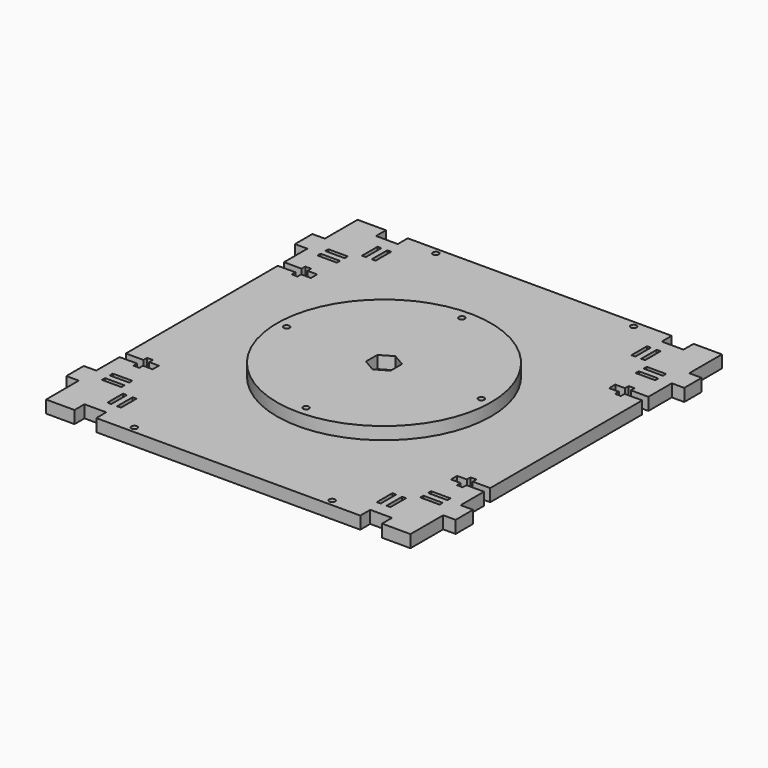
from build123d import *

# Parameters (mm, degrees)
F0_R     = 55
F0_R_2   = 1.5
F0_R_3   = 45
F1_DEPTH = 6.4
F2_DEPTH = 6
F0_R_4   = 85
F3_DEPTH = 6
F0_W     = 2
F0_H     = 10
F0_W_2   = 10
F0_H_2   = 2
F4_DEPTH = 6.4


with BuildPart() as f1:
    # F0 (on Top) → F1 (new body)
    with BuildSketch(Plane.XY):
        Circle(F0_R)
        with Locations((0, -50)):
            Circle(F0_R_2, mode=Mode.SUBTRACT)
        with Locations((-50, 0)):
            Circle(F0_R_2, mode=Mode.SUBTRACT)
        Circle(F0_R_3, mode=Mode.SUBTRACT)
        with Locations((50, 0)):
            Circle(F0_R_2, mode=Mode.SUBTRACT)
        with Locations((0, 50)):
            Circle(F0_R_2, mode=Mode.SUBTRACT)
        Circle(F0_R_3)
        Polygon((-6.35, 3.6661742094), (0, 7.3323484187), (6.35, 3.6661742094), (6.35, -3.6661742094), (0, -7.3323484187), (-6.35, -3.6661742094), align=None, mode=Mode.SUBTRACT)
    extrude(amount=F1_DEPTH)


with BuildPart() as f2:
    # F0 (on Top) → F2 (new body)
    with BuildSketch(Plane.XY):
        Circle(F0_R)
        with Locations((0, -50)):
            Circle(F0_R_2, mode=Mode.SUBTRACT)
        with Locations((-50, 0)):
            Circle(F0_R_2, mode=Mode.SUBTRACT)
        Circle(F0_R_3, mode=Mode.SUBTRACT)
        with Locations((50, 0)):
            Circle(F0_R_2, mode=Mode.SUBTRACT)
        with Locations((0, 50)):
            Circle(F0_R_2, mode=Mode.SUBTRACT)
    extrude(amount=F2_DEPTH)


with BuildPart() as f3:
    # F0 (on Top) → F3 (new body)
    with BuildSketch(Plane.XY):
        Circle(F0_R_4)
        Circle(F0_R, mode=Mode.SUBTRACT)
        Circle(F0_R)
        with Locations((0, -50)):
            Circle(F0_R_2, mode=Mode.SUBTRACT)
        with Locations((-50, 0)):
            Circle(F0_R_2, mode=Mode.SUBTRACT)
        Circle(F0_R_3, mode=Mode.SUBTRACT)
        with Locations((50, 0)):
            Circle(F0_R_2, mode=Mode.SUBTRACT)
        with Locations((0, 50)):
            Circle(F0_R_2, mode=Mode.SUBTRACT)
    extrude(amount=F3_DEPTH)


with BuildPart() as f4:
    # F0 (on Top) → F4 (new body)
    with BuildSketch(Plane.XY):
        Polygon((93.6, 78.994885087), (93.6, 100), (78.994885087, 100), (78.994885087, 93.6), (67.8103417158, 93.6), (67.8103417158, 100), (-67.8103417158, 100), (-67.8103417158, 93.6), (-78.994885087, 93.6), (-78.994885087, 100), (-93.6, 100), (-93.6, 78.994885087), (-100, 78.994885087), (-100, 67.8103417158), (-93.6, 67.8103417158), (-93.6, 52.7854223251), (-84.5765625, 52.7854223251), (-84.5765625, 55.1510473251), (-81.6, 55.1510473251), (-81.6, 52.7854223251), (-76.6, 52.7854223251), (-76.6, 48.7854223251), (-81.6, 48.7854223251), (-81.6, 46.4197973251), (-84.5765625, 46.4197973251), (-84.5765625, 48.7854223251), (-93.6, 48.7854223251), (-93.6, -48.7854223251), (-84.5765625, -48.7854223251), (-84.5765625, -46.4197973251), (-81.6, -46.4197973251), (-81.6, -48.7854223251), (-76.6, -48.7854223251), (-76.6, -52.7854223251), (-81.6, -52.7854223251), (-81.6, -55.1510473251), (-84.5765625, -55.1510473251), (-84.5765625, -52.7854223251), (-93.6, -52.7854223251), (-93.6, -67.8103417158), (-100, -67.8103417158), (-100, -78.994885087), (-93.6, -78.994885087), (-93.6, -100), (-78.994885087, -100), (-78.994885087, -93.6), (-67.8103417158, -93.6), (-67.8103417158, -100), (67.8103417158, -100), (67.8103417158, -93.6), (78.994885087, -93.6), (78.994885087, -100), (93.6, -100), (93.6, -78.994885087), (100, -78.994885087), (100, -67.8103417158), (93.6, -67.8103417158), (93.6, -52.7854223251), (84.5765625, -52.7854223251), (84.5765625, -55.1510473251), (81.6, -55.1510473251), (81.6, -52.7854223251), (76.6, -52.7854223251), (76.6, -48.7854223251), (81.6, -48.7854223251), (81.6, -46.4197973251), (84.5765625, -46.4197973251), (84.5765625, -48.7854223251), (93.6, -48.7854223251), (93.6, 48.7854223251), (84.5765625, 48.7854223251), (84.5765625, 46.4197973251), (81.6, 46.4197973251), (81.6, 48.7854223251), (76.6, 48.7854223251), (76.6, 52.7854223251), (81.6, 52.7854223251), (81.6, 55.1510473251), (84.5765625, 55.1510473251), (84.5765625, 52.7854223251), (93.6, 52.7854223251), (93.6, 67.8103417158), (100, 67.8103417158), (100, 78.994885087), align=None)
        with Locations((-50.7854223251, -96.8)):
            Circle(F0_R_2, mode=Mode.SUBTRACT)
        with Locations((-71.6977112889, -81.7467170954)):
            Rectangle(F0_W, F0_H, mode=Mode.SUBTRACT)
        with Locations((-66.6977112889, -81.7467170954)):
            Rectangle(F0_W, F0_H, mode=Mode.SUBTRACT)
        with Locations((-81.7467170954, -71.6977112889)):
            Rectangle(F0_W_2, F0_H_2, mode=Mode.SUBTRACT)
        with Locations((-81.7467170954, -66.6977112889)):
            Rectangle(F0_W_2, F0_H_2, mode=Mode.SUBTRACT)
        with Locations((50.7854223251, -96.8)):
            Circle(F0_R_2, mode=Mode.SUBTRACT)
        with Locations((66.6977112889, -81.7467170954)):
            Rectangle(F0_W, F0_H, mode=Mode.SUBTRACT)
        with Locations((71.6977112889, -81.7467170954)):
            Rectangle(F0_W, F0_H, mode=Mode.SUBTRACT)
        with Locations((81.7467170954, -71.6977112889)):
            Rectangle(F0_W_2, F0_H_2, mode=Mode.SUBTRACT)
        with Locations((81.7467170954, -66.6977112889)):
            Rectangle(F0_W_2, F0_H_2, mode=Mode.SUBTRACT)
        with Locations((-81.7467170954, 66.6977112889)):
            Rectangle(F0_W_2, F0_H_2, mode=Mode.SUBTRACT)
        with Locations((-81.7467170954, 71.6977112889)):
            Rectangle(F0_W_2, F0_H_2, mode=Mode.SUBTRACT)
        with Locations((-71.6977112889, 81.7467170954)):
            Rectangle(F0_W, F0_H, mode=Mode.SUBTRACT)
        with Locations((-66.6977112889, 81.7467170954)):
            Rectangle(F0_W, F0_H, mode=Mode.SUBTRACT)
        with Locations((-50.7854223251, 96.8)):
            Circle(F0_R_2, mode=Mode.SUBTRACT)
        Circle(F0_R_4, mode=Mode.SUBTRACT)
        with Locations((81.7467170954, 66.6977112889)):
            Rectangle(F0_W_2, F0_H_2, mode=Mode.SUBTRACT)
        with Locations((81.7467170954, 71.6977112889)):
            Rectangle(F0_W_2, F0_H_2, mode=Mode.SUBTRACT)
        with Locations((66.6977112889, 81.7467170954)):
            Rectangle(F0_W, F0_H, mode=Mode.SUBTRACT)
        with Locations((71.6977112889, 81.7467170954)):
            Rectangle(F0_W, F0_H, mode=Mode.SUBTRACT)
        with Locations((50.7854223251, 96.8)):
            Circle(F0_R_2, mode=Mode.SUBTRACT)
        Circle(F0_R_4)
        Circle(F0_R, mode=Mode.SUBTRACT)
        Circle(F0_R)
        with Locations((0, -50)):
            Circle(F0_R_2, mode=Mode.SUBTRACT)
        with Locations((-50, 0)):
            Circle(F0_R_2, mode=Mode.SUBTRACT)
        Circle(F0_R_3, mode=Mode.SUBTRACT)
        with Locations((50, 0)):
            Circle(F0_R_2, mode=Mode.SUBTRACT)
        with Locations((0, 50)):
            Circle(F0_R_2, mode=Mode.SUBTRACT)
    extrude(amount=F4_DEPTH)


with BuildPart() as f1_1:
    # F5: moved
    add(f1.part.moved(Location((0, 0, 6.4))))


solid = Compound([f2.part, f3.part, f4.part, f1_1.part])
